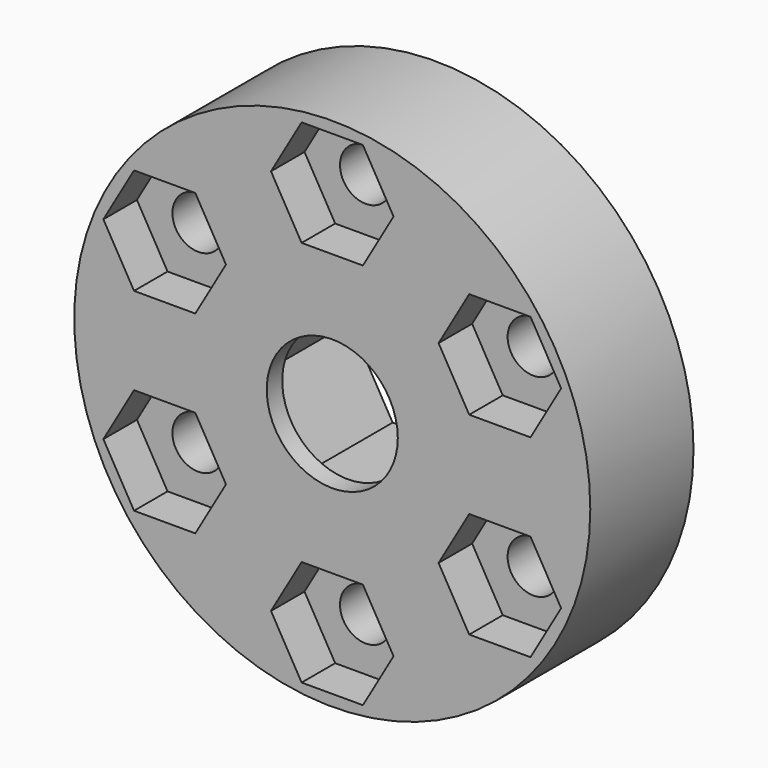
from build123d import *

# Parameters (mm, degrees)
F0_R            = 20
F1_DEPTH        = 10
F3_DEPTH        = 8.5
F4_R            = 2
F5_DEPTH        = 10.001
F5_COPIES_COUNT = 6
F7_DEPTH        = 3.25
F7_COPIES_COUNT = 6
F8_R            = 5.08
F9_DEPTH        = 10.001


# Not quite as in the source:
# - a pattern or mirror of a feature is missing from the dataset's text; its kind, count and spacing are read off the source's solid


with BuildPart() as f1:
    # F0 (on Front) → F1 (new body)
    with BuildSketch(Plane.XZ):
        Circle(F0_R)
    extrude(amount=F1_DEPTH)

    # F2 (on face) → F3 (cut)
    with BuildSketch(Plane(origin=(0, 0, 0), x_dir=(-1, 0, 0), z_dir=(0, 1, 0))):
        Polygon((3.3197640478, 5.75), (-3.3197640478, 5.75), (-6.6395280957, 0), (-3.3197640478, -5.75), (3.3197640478, -5.75), (6.6395280957, 0), align=None)
    extrude(amount=-F3_DEPTH, mode=Mode.SUBTRACT)

    # F4 (on face) → F5 (cut, through all)
    with BuildSketch(Plane.XZ.offset(10)):
        with Locations((0, 15)):
            Circle(F4_R)
    f5 = extrude(amount=-F5_DEPTH, mode=Mode.SUBTRACT)

    # F5_copies: F5 ×6 about axis
    f5_copies_axis = Axis((0, 0, 0), (0, 1, 0))
    for i in range(1, F5_COPIES_COUNT):
        add(f5.rotate(f5_copies_axis, i * 360 / F5_COPIES_COUNT), mode=Mode.SUBTRACT)

    # F6 (on face) → F7 (cut)
    with BuildSketch(Plane.XZ.offset(10)):
        Polygon((2.375, 19.113620668), (-2.375, 19.113620668), (-4.75, 15), (-2.375, 10.886379332), (2.375, 10.886379332), (4.75, 15), align=None)
    f7 = extrude(amount=-F7_DEPTH, mode=Mode.SUBTRACT)

    # F7_copies: F7 ×6 about axis
    f7_copies_axis = Axis((0, 0, 0), (0, 1, 0))
    for i in range(1, F7_COPIES_COUNT):
        add(f7.rotate(f7_copies_axis, i * 360 / F7_COPIES_COUNT), mode=Mode.SUBTRACT)

    # F8 (on face) → F9 (cut, through all)
    with BuildSketch(Plane.XZ.offset(10)):
        Circle(F8_R)
    extrude(amount=-F9_DEPTH, mode=Mode.SUBTRACT)


solid = f1.part
